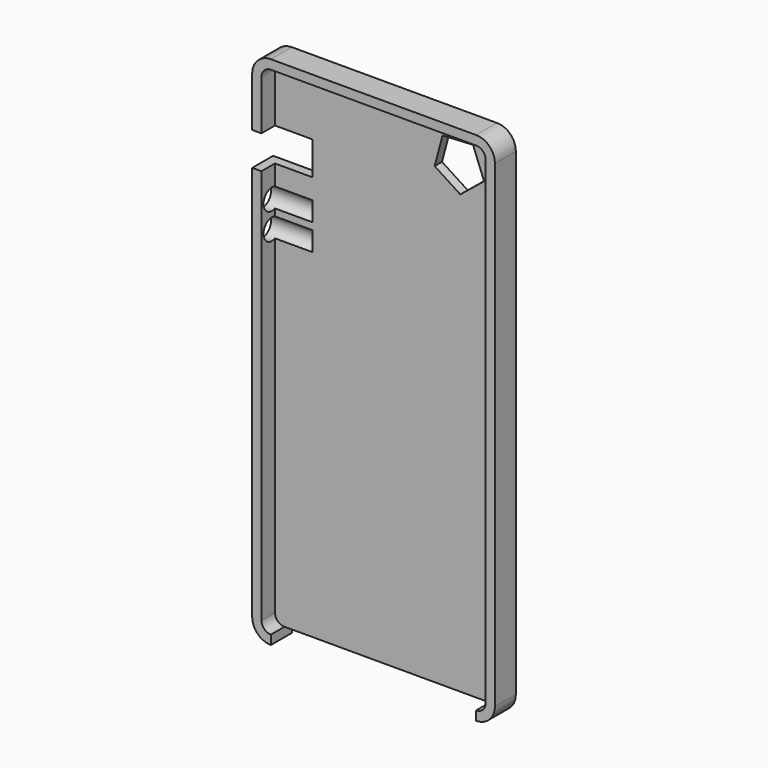
from build123d import *

# Parameters (mm, degrees)
F0_W      = 65.8367946744
F0_H      = 139.9032026529
F1_DEPTH  = 3.55
F2_R      = 5.08
F3_T      = -2.5
F5_DEPTH  = 12.7
F6_W      = 55.6767946744
F6_H      = 7.1
F7_DEPTH  = 2.5019
F8_W      = 7.1
F8_H      = 9.0527832508
F8_R      = 2.8313125725
F8_R_2    = 2.8285937047
F9_DEPTH  = 12.7
F10_DEPTH = 0.5


# Not quite as in the source:
# - a feature names something its author has since deleted; it is built from what else it names


with BuildPart() as f1:
    # F0 (on Front) → F1 (new body, symmetric)
    with BuildSketch(Plane.XZ):
        Rectangle(F0_W, F0_H)
    extrude(amount=F1_DEPTH, both=True)

    # F2
    f2_edges = [f1.edges().sort_by_distance(p)[0] for p in [
        (-32.918397, 0, 69.951601),
        (32.918397, 0, 69.951601),
        (-32.918397, 0, -69.951601),
        (32.918397, 0, -69.951601),
    ]]
    fillet(f2_edges, radius=F2_R)

    # F3
    f3_openings = [f1.faces().sort_by_distance(p)[0] for p in [
        (0, -3.55, 0),
    ]]
    offset(amount=F3_T, openings=f3_openings)

    # F4 (on Front) → F5 (cut, symmetric)
    with BuildSketch(Plane.XZ):
        Polygon((12.9001184621, 55.8146053817), (19.8599101564, 51.3060083088), (26.2985346927, 56.5319304354), (23.3180318028, 64.2703250051), (15.0373551768, 63.8269937409), align=None)
    extrude(amount=F5_DEPTH, both=True, mode=Mode.SUBTRACT)

    # F6 (on face) → F7 (cut, symmetric)
    with BuildSketch(Plane(origin=(0, 0, -69.9516013265), x_dir=(1, 0, 0), z_dir=(0, 0, -1))):
        Rectangle(F6_W, F6_H)
    extrude(amount=F7_DEPTH, both=True, mode=Mode.SUBTRACT)

    # F8 (on face) → F9 (cut, symmetric)
    with BuildSketch(Plane(origin=(-32.9183973372, 0, 0), x_dir=(0, -1, 0), z_dir=(-1, 0, 0))):
        with Locations((0, 46.8815155327)):
            Rectangle(F8_W, F8_H)
        with Locations((0, 34.2498570681)):
            Circle(F8_R)
        with Locations((0, 27.1013174206)):
            Circle(F8_R_2)
    extrude(amount=F9_DEPTH, both=True, mode=Mode.SUBTRACT)

    # F8 (on face) → F10 (cut, symmetric)
    with BuildSketch(Plane(origin=(-32.9183973372, 0, 0), x_dir=(0, -1, 0), z_dir=(-1, 0, 0))):
        with Locations((0, 46.8815155327)):
            Rectangle(F8_W, F8_H)
        with Locations((0, 34.2498570681)):
            Circle(F8_R)
        with Locations((0, 27.1013174206)):
            Circle(F8_R_2)
    extrude(amount=F10_DEPTH, both=True, mode=Mode.SUBTRACT)


solid = f1.part
